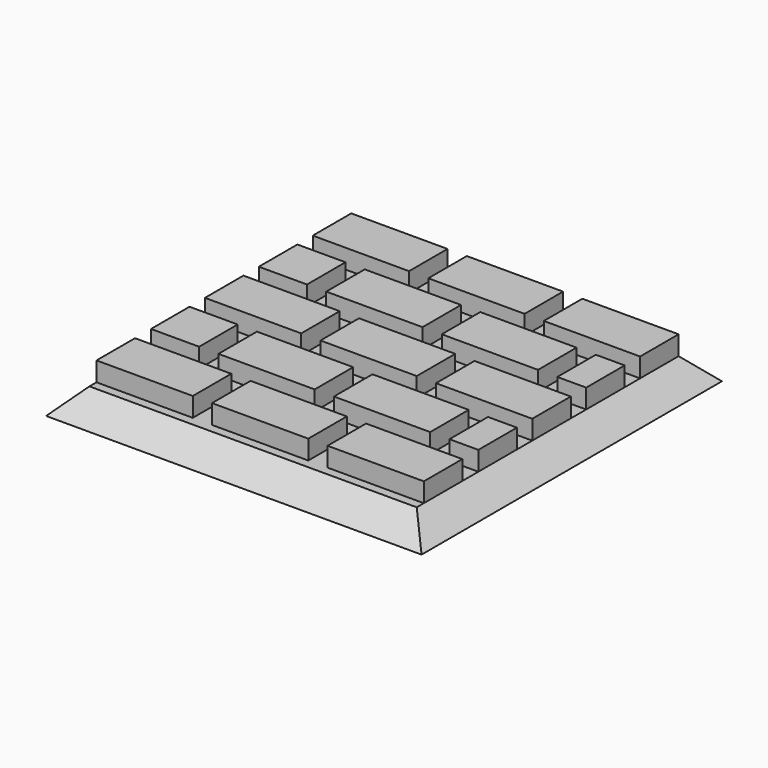
from build123d import *

# Parameters (mm, degrees)
F0_W     = 49.53
F0_H     = 49.53
F1_DEPTH = 3.175
F2_SIZE  = 3.17499
F3_W     = 3.81
F3_H     = 6.35
F3_W_2   = 12.7
F3_W_3   = 6.35
F3_W_4   = 12.7000000036
F3_W_5   = 3.8100000384
F3_W_6   = 12.7000000384
F4_DEPTH = 2.54


# Not quite as in the source:
# - a fillet or chamfer is up to 0.001 mm smaller than in the source, because OpenCascade refuses the exact size


with BuildPart() as f1:
    # F0 (on Top) → F1 (new body)
    with BuildSketch(Plane.XY):
        with Locations((24.765, 24.765)):
            Rectangle(F0_W, F0_H)
    extrude(amount=F1_DEPTH)

    # F2 (size 3.175 in the source; OpenCascade refuses exactly that, so slightly less here)
    f2_edges = [f1.edges().sort_by_distance(p)[0] for p in [
        (0, 24.765, 3.175),
        (24.765, 0, 3.175),
        (49.53, 24.765, 3.175),
        (24.765, 49.53, 3.175),
    ]]
    chamfer(f2_edges, length=F2_SIZE)

    # F3 (on face) → F4 (join)
    with BuildSketch(Plane.XY.offset(3.175)):
        with Locations((44.45, 34.29)):
            Rectangle(F3_W, F3_H)
        with Locations((9.525, 43.18)):
            Rectangle(F3_W_2, F3_H)
        with Locations((9.5249999653, 25.4)):
            Rectangle(F3_W_2, F3_H)
        with Locations((24.765, 43.18)):
            Rectangle(F3_W_2, F3_H)
        with Locations((6.3499999653, 16.51)):
            Rectangle(F3_W_3, F3_H)
        with Locations((40.005, 43.18)):
            Rectangle(F3_W_2, F3_H)
        with Locations((33.6549999616, 16.51)):
            Rectangle(F3_W_2, F3_H)
        with Locations((9.525, 7.5206288218)):
            Rectangle(F3_W_2, F3_H)
        with Locations((6.35, 34.29)):
            Rectangle(F3_W_3, F3_H)
        with Locations((24.7649999653, 25.4)):
            Rectangle(F3_W_2, F3_H)
        with Locations((40.0049999982, 7.5206288218)):
            Rectangle(F3_W_4, F3_H)
        with Locations((18.415, 34.29)):
            Rectangle(F3_W_2, F3_H)
        with Locations((18.4149999616, 16.51)):
            Rectangle(F3_W_2, F3_H)
        with Locations((44.4499999808, 16.51)):
            Rectangle(F3_W_5, F3_H)
        with Locations((33.655, 34.29)):
            Rectangle(F3_W_2, F3_H)
        with Locations((40.0049999808, 25.4)):
            Rectangle(F3_W_6, F3_H)
        with Locations((24.765, 7.5206288218)):
            Rectangle(F3_W_2, F3_H)
    extrude(amount=F4_DEPTH)


solid = f1.part
